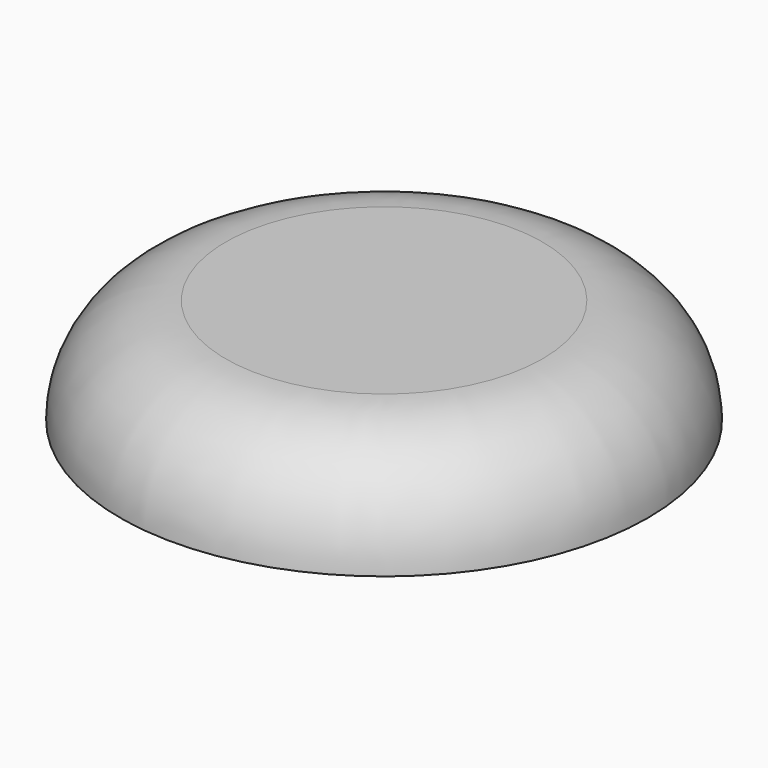
from build123d import *

# Parameters (mm, degrees)
F0_R     = 15
F1_DEPTH = 6
F2_R     = 5.99999
F3_T     = 2.5


# Not quite as in the source:
# - a fillet or chamfer is up to 0.001 mm smaller than in the source, because OpenCascade refuses the exact size
# - a shell that OpenCascade refuses in one call is made with other operations: the cavity is built on its own and cut out


with BuildPart() as f1:
    # F0 (on Top) → F1 (new body)
    with BuildSketch(Plane.XY):
        Circle(F0_R)
    extrude(amount=F1_DEPTH)

    # F2 (radius 6 in the source; OpenCascade refuses exactly that, so slightly less here)
    f2_edges = [f1.edges().sort_by_distance(p)[0] for p in [
        (-15, 0, 6),
    ]]
    fillet(f2_edges, radius=F2_R)

    # F3: shell of thickness 2.5, made by hand


with BuildPart() as f3_core1:
    # F3_t2: copy of F1
    add(f1.part)

    # the walls: a layer under each face that stays
    f3_faces = [f3_core1.faces().sort_by_distance(p)[0] for p in [
        (-15, 0, 5e-06),
        (-13.2426436161, 0, 4.2426436161),
        (0, 0, 6),
    ]]
    thicken(f3_faces, amount=-F3_T, mode=Mode.SUBTRACT)


with BuildPart() as f1_1:
    add(f1.part)

    # what is left inside the walls is the cavity
    f3_cavity = [f3_core1.part.solids().sort_by_distance(p)[0] for p in [
        (0, -4.166667, 0.025),
    ]]
    add(f3_cavity, mode=Mode.SUBTRACT)


solid = f1_1.part
